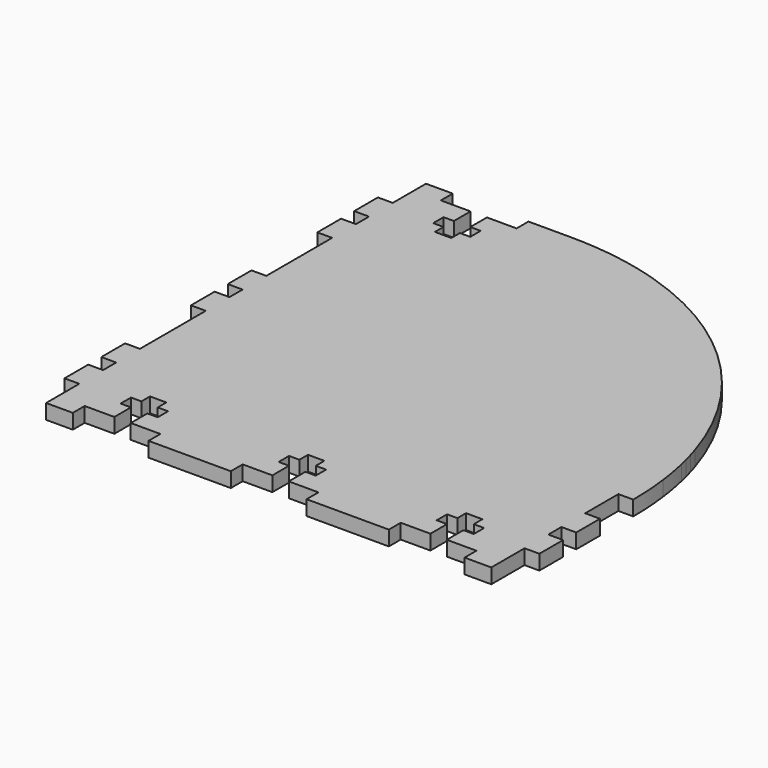
from build123d import *

# Parameters (mm, degrees)
F0_W     = 3.175
F0_H     = 6.35
F0_W_2   = 3.5052
F0_H_2   = 4.445
F0_H_3   = 2.778125
F0_W_3   = 2.21615
F0_H_4   = 2.301875
F1_DEPTH = 3.175


with BuildPart() as f1:
    # F0 (on Top) → F1 (new body)
    with BuildSketch(Plane.XY):
        with BuildLine():
            Line((-39.248683933, 94.5405161858), (-44.963683933, 94.5405161858))
            Line((-44.963683933, 94.5405161858), (-44.963683933, 85.6505161858))
            Line((-44.963683933, 85.6505161858), (-44.963683933, 79.3005161858))
            Line((-44.963683933, 79.3005161858), (-44.963683933, 75.7953161858))
            Line((-44.963683933, 75.7953161858), (-44.963683933, 69.4453161858))
            Line((-44.963683933, 69.4453161858), (-44.963683933, 51.8431161858))
            Line((-44.963683933, 51.8431161858), (-44.963683933, 45.4931161858))
            Line((-44.963683933, 45.4931161858), (-44.963683933, 43.7405161858))
            Line((-44.963683933, 43.7405161858), (50.286316067, 43.7405161858))
            Line((50.286316067, 43.7405161858), (50.286316067, 45.4931161858))
            Line((50.286316067, 45.4931161858), (50.286316067, 47.4018817204))
            ThreePointArc((50.286316067, 47.4018817204), (33.6573996556, 74.7365997743), (6.3226816016, 91.3655161858))
            Line((6.3226816016, 91.3655161858), (4.413916067, 91.3655161858))
            Line((4.413916067, 91.3655161858), (4.413916067, 86.9205161858))
            Line((4.413916067, 86.9205161858), (6.630066067, 86.9205161858))
            Line((6.630066067, 86.9205161858), (6.630066067, 84.1423911858))
            Line((6.630066067, 84.1423911858), (4.413916067, 84.1423911858))
            Line((4.413916067, 84.1423911858), (4.413916067, 81.8405161858))
            Line((4.413916067, 81.8405161858), (0.908716067, 81.8405161858))
            Line((0.908716067, 81.8405161858), (0.908716067, 84.1423911858))
            Line((0.908716067, 84.1423911858), (-1.307433933, 84.1423911858))
            Line((-1.307433933, 84.1423911858), (-1.307433933, 86.9205161858))
            Line((-1.307433933, 86.9205161858), (0.908716067, 86.9205161858))
            Line((0.908716067, 86.9205161858), (0.908716067, 91.3655161858))
            Line((0.908716067, 91.3655161858), (-5.441283933, 91.3655161858))
            Line((-5.441283933, 91.3655161858), (-5.441283933, 93.9768813524))
            ThreePointArc((-5.441283933, 93.9768813524), (-9.7882773782, 94.3994603443), (-14.153483933, 94.5405161858))
            Line((-14.153483933, 94.5405161858), (-23.043483933, 94.5405161858))
            Line((-23.043483933, 94.5405161858), (-23.043483933, 91.3655161858))
            Line((-23.043483933, 91.3655161858), (-29.393483933, 91.3655161858))
            Line((-29.393483933, 91.3655161858), (-29.393483933, 86.9205161858))
            Line((-29.393483933, 86.9205161858), (-27.177333933, 86.9205161858))
            Line((-27.177333933, 86.9205161858), (-27.177333933, 84.1423911858))
            Line((-27.177333933, 84.1423911858), (-29.393483933, 84.1423911858))
            Line((-29.393483933, 84.1423911858), (-29.393483933, 81.8405161858))
            Line((-29.393483933, 81.8405161858), (-32.898683933, 81.8405161858))
            Line((-32.898683933, 81.8405161858), (-32.898683933, 84.1423911858))
            Line((-32.898683933, 84.1423911858), (-35.114833933, 84.1423911858))
            Line((-35.114833933, 84.1423911858), (-35.114833933, 86.9205161858))
            Line((-35.114833933, 86.9205161858), (-32.898683933, 86.9205161858))
            Line((-32.898683933, 86.9205161858), (-32.898683933, 91.3655161858))
            Line((-32.898683933, 91.3655161858), (-39.248683933, 91.3655161858))
            Line((-39.248683933, 91.3655161858), (-39.248683933, 94.5405161858))
        make_face()
        with Locations((-46.551183933, 82.4755161858)):
            Rectangle(F0_W, F0_H)
        with Locations((-46.551183933, 72.6203161858)):
            Rectangle(F0_W, F0_H)
        with Locations((-46.551183933, 48.6681161858)):
            Rectangle(F0_W, F0_H)
        with BuildLine():
            ThreePointArc((0.908716067, 92.8415057221), (-2.252736339, 93.4849633701), (-5.441283933, 93.9768813524))
            Line((-5.441283933, 93.9768813524), (-5.441283933, 91.3655161858))
            Line((-5.441283933, 91.3655161858), (0.908716067, 91.3655161858))
            Line((0.908716067, 91.3655161858), (0.908716067, 92.8415057221))
        make_face()
        with BuildLine():
            ThreePointArc((4.413916067, 91.9411976981), (2.6673405912, 92.4148071961), (0.908716067, 92.8415057221))
            Line((0.908716067, 92.8415057221), (0.908716067, 91.3655161858))
            Line((0.908716067, 91.3655161858), (4.413916067, 91.3655161858))
            Line((4.413916067, 91.3655161858), (4.413916067, 91.9411976981))
        make_face()
        Polygon((50.286316067, 43.7405161858), (-44.963683933, 43.7405161858), (-44.963683933, 41.9879161858), (-44.963683933, 35.6379161858), (-44.963683933, 18.0357161858), (-44.963683933, 11.6857161858), (-44.963683933, 8.1805161858), (-44.963683933, 1.8305161858), (-44.963683933, -7.0594838142), (-39.248683933, -7.0594838142), (-39.248683933, -3.8844838142), (-32.898683933, -3.8844838142), (-32.898683933, 0.5605161858), (-35.114833933, 0.5605161858), (-35.114833933, 3.3386411858), (-32.898683933, 3.3386411858), (-32.898683933, 5.6405161858), (-29.393483933, 5.6405161858), (-29.393483933, 3.3386411858), (-27.177333933, 3.3386411858), (-27.177333933, 0.5605161858), (-29.393483933, 0.5605161858), (-29.393483933, -3.8844838142), (-23.043483933, -3.8844838142), (-23.043483933, -7.0594838142), (-5.441283933, -7.0594838142), (-5.441283933, -3.8844838142), (0.908716067, -3.8844838142), (0.908716067, 0.5605161858), (-1.307433933, 0.5605161858), (-1.307433933, 3.3386411858), (0.908716067, 3.3386411858), (0.908716067, 5.6405161858), (4.413916067, 5.6405161858), (4.413916067, 3.3386411858), (6.630066067, 3.3386411858), (6.630066067, 0.5605161858), (4.413916067, 0.5605161858), (4.413916067, -3.8844838142), (10.763916067, -3.8844838142), (10.763916067, -7.0594838142), (28.366116067, -7.0594838142), (28.366116067, -3.8844838142), (34.716116067, -3.8844838142), (34.716116067, 0.5605161858), (32.499966067, 0.5605161858), (32.499966067, 3.3386411858), (34.716116067, 3.3386411858), (34.716116067, 5.6405161858), (38.221316067, 5.6405161858), (38.221316067, 3.3386411858), (40.437466067, 3.3386411858), (40.437466067, 0.5605161858), (38.221316067, 0.5605161858), (38.221316067, -3.8844838142), (44.571316067, -3.8844838142), (44.571316067, -7.0594838142), (50.286316067, -7.0594838142), (50.286316067, 1.8305161858), (50.286316067, 8.1805161858), (50.286316067, 11.6857161858), (50.286316067, 18.0357161858), (50.286316067, 26.9257161858), (50.286316067, 35.6379161858), (50.286316067, 41.9879161858), align=None)
        with Locations((-46.551183933, 38.8129161858)):
            Rectangle(F0_W, F0_H)
        with Locations((2.661316067, 89.1430161858)):
            Rectangle(F0_W_2, F0_H_2)
        with BuildLine():
            ThreePointArc((6.3226816016, 91.3655161858), (5.3704207665, 91.6603925526), (4.413916067, 91.9411976981))
            Line((4.413916067, 91.9411976981), (4.413916067, 91.3655161858))
            Line((4.413916067, 91.3655161858), (6.3226816016, 91.3655161858))
        make_face()
        with BuildLine():
            Line((50.286316067, 45.4931161858), (50.286316067, 43.7405161858))
            Line((50.286316067, 43.7405161858), (51.3371541766, 43.7405161858))
            ThreePointArc((51.3371541766, 43.7405161858), (51.1054596409, 44.6184113637), (50.8619975793, 45.4931161858))
            Line((50.8619975793, 45.4931161858), (50.286316067, 45.4931161858))
        make_face()
        with BuildLine():
            Line((51.3371541766, 43.7405161858), (50.286316067, 43.7405161858))
            Line((50.286316067, 43.7405161858), (50.286316067, 41.9879161858))
            Line((50.286316067, 41.9879161858), (51.7623056033, 41.9879161858))
            ThreePointArc((51.7623056033, 41.9879161858), (51.5555733449, 42.8656337101), (51.3371541766, 43.7405161858))
        make_face()
        with Locations((2.661316067, 85.5314536858)):
            Rectangle(F0_W_2, F0_H_3)
        with Locations((-0.199358933, 85.5314536858)):
            Rectangle(F0_W_3, F0_H_3)
        with BuildLine():
            Line((51.7623056033, 41.9879161858), (50.286316067, 41.9879161858))
            Line((50.286316067, 41.9879161858), (50.286316067, 35.6379161858))
            Line((50.286316067, 35.6379161858), (52.8976812336, 35.6379161858))
            ThreePointArc((52.8976812336, 35.6379161858), (52.4057632513, 38.8264637797), (51.7623056033, 41.9879161858))
        make_face()
        with BuildLine():
            Line((50.286316067, 47.4018817204), (50.286316067, 45.4931161858))
            Line((50.286316067, 45.4931161858), (50.8619975793, 45.4931161858))
            ThreePointArc((50.8619975793, 45.4931161858), (50.5811924339, 46.4496208852), (50.286316067, 47.4018817204))
        make_face()
        with Locations((-46.551183933, 14.8607161858)):
            Rectangle(F0_W, F0_H)
        with Locations((5.521991067, 85.5314536858)):
            Rectangle(F0_W_3, F0_H_3)
        with Locations((2.661316067, 82.9914536858)):
            Rectangle(F0_W_2, F0_H_4)
        with BuildLine():
            Line((52.8976812336, 35.6379161858), (50.286316067, 35.6379161858))
            Line((50.286316067, 35.6379161858), (50.286316067, 26.9257161858))
            Line((50.286316067, 26.9257161858), (53.461316067, 26.9257161858))
            ThreePointArc((53.461316067, 26.9257161858), (53.3202602255, 31.2909227406), (52.8976812336, 35.6379161858))
        make_face()
        with Locations((-46.551183933, 5.0055161858)):
            Rectangle(F0_W, F0_H)
        with Locations((51.873816067, 14.8607161858)):
            Rectangle(F0_W, F0_H)
        with Locations((51.873816067, 5.0055161858)):
            Rectangle(F0_W, F0_H)
    extrude(amount=F1_DEPTH)


solid = f1.part
